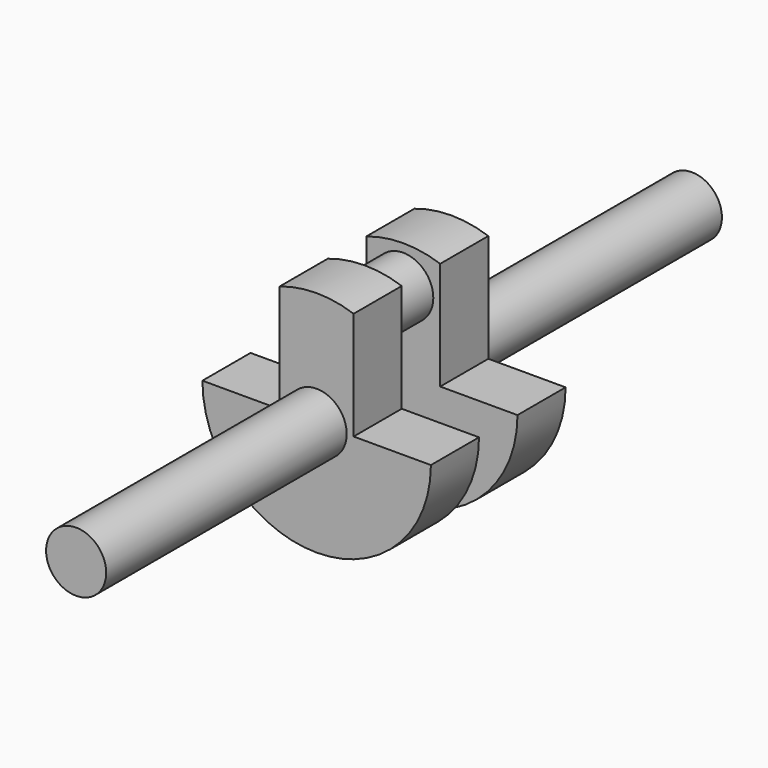
from build123d import *

# Parameters (mm, degrees)
F1_DEPTH = 2.5
F2_R     = 2.5
F4_DEPTH = 14
F5_R     = 2.5
F6_DEPTH = 30
F7_R     = 2.5
F8_DEPTH = 30


# Not quite as in the source:
# - a feature names something its author has since deleted; it is built from what else it names


with BuildPart() as f1:
    # F0 (on Front) → F1 (new body, symmetric)
    with BuildSketch(Plane.XZ):
        with BuildLine():
            ThreePointArc((-3.0750329511, -8.9885578571), (0, -9.5), (3.0750329511, -8.9885578571))
            Line((3.0750329511, -8.9885578571), (3.0750329511, 0))
            Line((3.0750329511, 0), (3.0750329511, 8.9885578571))
            ThreePointArc((3.0750329511, 8.9885578571), (0, 9.5), (-3.0750329511, 8.9885578571))
            Line((-3.0750329511, 8.9885578571), (-3.0750329511, 0))
            Line((-3.0750329511, 0), (-3.0750329511, -8.9885578571))
        make_face()
        with BuildLine():
            ThreePointArc((-9.5, 0), (-7.7286096109, -5.5243636269), (-3.0750329511, -8.9885578571))
            Line((-3.0750329511, -8.9885578571), (-3.0750329511, 0))
            Line((-3.0750329511, 0), (-9.5, 0))
        make_face()
        with BuildLine():
            Line((3.0750329511, 0), (3.0750329511, -8.9885578571))
            ThreePointArc((3.0750329511, -8.9885578571), (7.7286096109, -5.5243636269), (9.5, 0))
            Line((9.5, 0), (3.0750329511, 0))
        make_face()
    extrude(amount=F1_DEPTH, both=True)


with BuildPart() as f3_1:
    # F3: copy of F1
    add(f1.part.moved(Location((0, 9, 0))))


with BuildPart() as f1_1:
    add(f1.part)

    add(f3_1.part)  # F4 merges F3_1
    # F2 (on face) → F4 (join, through all)
    with BuildSketch(Plane.XZ.offset(2.5)):
        with Locations((0, 6.3)):
            Circle(F2_R)
    extrude(amount=-F4_DEPTH)

    # F5 (on face) → F6 (join)
    with BuildSketch(Plane(origin=(0, 2.5, 0), x_dir=(-1, 0, 0), z_dir=(0, 1, 0))):
        Circle(F5_R)
    extrude(amount=-F6_DEPTH)

    # F7 (on face) → F8 (join)
    with BuildSketch(Plane.XZ.offset(-6.5)):
        Circle(F7_R)
    extrude(amount=-F8_DEPTH)


solid = f1_1.part
